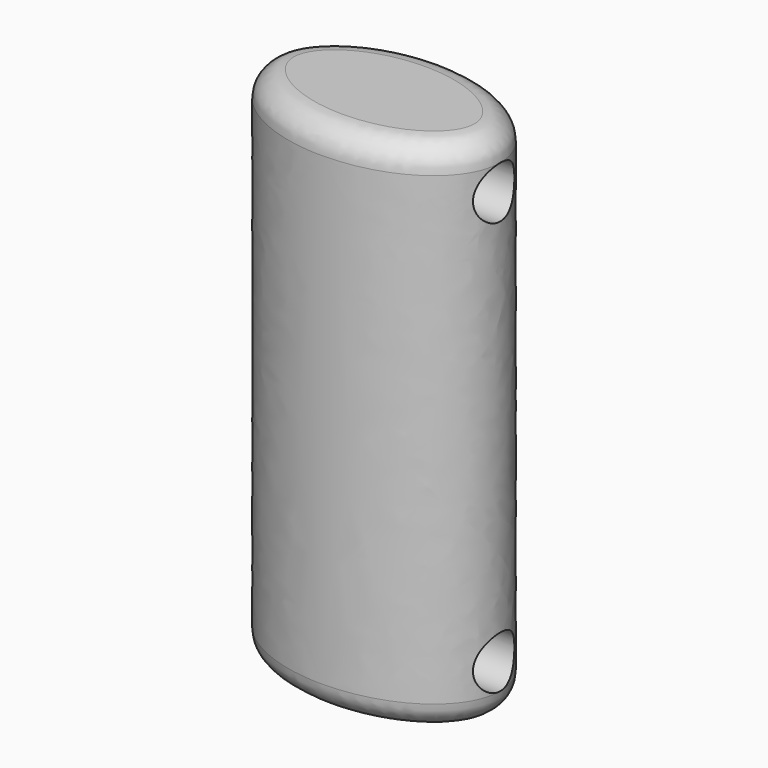
from build123d import *

# Parameters (mm, degrees)
F1_DEPTH = 100
F2_R     = 5
F3_DEPTH = 25
F4_R     = 4.99999


# Not quite as in the source:
# - a fillet or chamfer is up to 0.001 mm smaller than in the source, because OpenCascade refuses the exact size


with BuildPart() as f1:
    # F0 (on Top) → F1 (new body)
    with BuildSketch(Plane.XY):
        with BuildLine():
            add(Edge.make_bspline(
                [(0, -15), (38.9711431703, -15), (19.4855715851, 7.5), (0, 30), (-19.4855715851, 7.5), (-38.9711431703, -15), (0, -15)],
                knots=[4.7123889804, 4.7123889804, 4.7123889804, 6.8067840828, 6.8067840828, 8.9011791852, 8.9011791852, 10.9955742876, 10.9955742876, 10.9955742876], degree=2, weights=[1, 0.5, 1, 0.5, 1, 0.5, 1]))
        make_face()
    extrude(amount=F1_DEPTH)

    # F2 (on Right) → F3 (cut, symmetric)
    with BuildSketch(Plane.YZ):
        with Locations((0, 90)):
            Circle(F2_R)
        with Locations((0, 10)):
            Circle(F2_R)
    extrude(amount=F3_DEPTH, both=True, mode=Mode.SUBTRACT)

    # F4 (radius 5 in the source; OpenCascade refuses exactly that, so slightly less here)
    f4_edges = [f1.edges().sort_by_distance(p)[0] for p in [
        (0, 15, 100),
        (0, 15, 0),
    ]]
    fillet(f4_edges, radius=F4_R)


solid = f1.part
